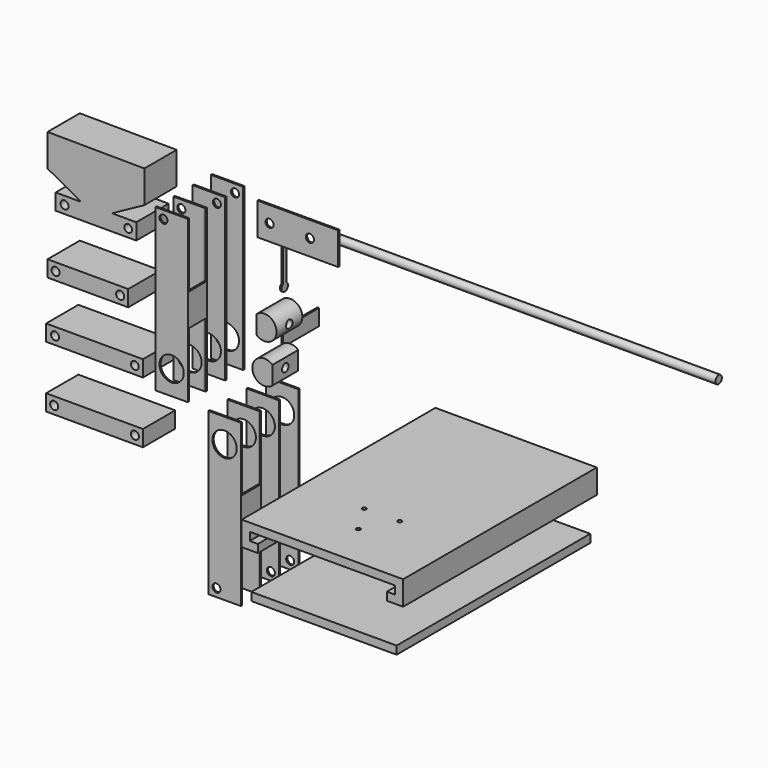
from build123d import *

# Parameters (mm, degrees)
F1_DEPTH  = 100
F2_R      = 7.5
F2_R_2    = 2.5
F3_DEPTH  = 15.001
F4_W      = 13
F4_H      = 40
F5_DEPTH  = 20.1627097718
F6_DEPTH  = 100
F7_R      = 7.5
F7_R_2    = 2.5
F8_DEPTH  = 16.001
F9_W      = 14
F9_H      = 40
F10_DEPTH = 20.1691592966
F11_W     = 50
F11_H     = 20
F11_R     = 2.5
F12_DEPTH = 1
F13_R     = 2.5
F13_R_2   = 7.5
F14_DEPTH = 45.1330833913
F15_R     = 7.5
F15_R_2   = 2.5
F16_DEPTH = 46.1330833913
F17_W     = 14
F17_H     = 40
F18_DEPTH = 53.5847666336
F19_W     = 13
F19_H     = 40
F20_DEPTH = 25
F22_DEPTH = 20
F23_R     = 2.5
F24_DEPTH = 250
F25_W     = 50
F25_H     = 10
F25_R     = 2.5
F26_DEPTH = 25
F25_R_2   = 2.4144593705
F25_W_2   = 60
F27_DEPTH = 25
F28_R     = 2.5
F29_DEPTH = 136.2251037518
F30_R     = 2.5
F31_DEPTH = 214.5146418358
F33_DEPTH = 1
F34_W     = 1
F34_H     = 10
F35_DEPTH = 25
F37_DEPTH = 150
F38_R     = 1.25
F39_DEPTH = 94.0357944536


# Not quite as in the source:
# - a feature names something its author has since deleted; it is built from what else it names


with BuildPart() as f1:
    # F0 (on Top) → F1 (new body)
    with BuildSketch(Plane.XY):
        Polygon((0, 14), (0, 15), (-20, 15), (-20, 0), (0, 0), (0, 1), (-19, 1), (-19, 14), align=None)
    extrude(amount=F1_DEPTH)

    # F2 (on face) → F3 (cut, through all)
    with BuildSketch(Plane.XZ):
        with Locations((-10, 15)):
            Circle(F2_R)
        with Locations((-5, 95)):
            Circle(F2_R_2)
    extrude(amount=-F3_DEPTH, mode=Mode.SUBTRACT)

    # F4 (on face) → F5 (cut, through all)
    with BuildSketch(Plane(origin=(-20, 0, 0), x_dir=(0, -1, 0), z_dir=(-1, 0, 0))):
        with Locations((-7.5, 20)):
            Rectangle(F4_W, F4_H)
        with Locations((-7.5, 80)):
            Rectangle(F4_W, F4_H)
    extrude(amount=-F5_DEPTH, mode=Mode.SUBTRACT)


with BuildPart() as f1b:
    # F0 (on Top) → F1, piece 2 (new body)
    with BuildSketch(Plane.XY):
        Polygon((0.051417134, -13.985459061), (-19.9480422158, -14.1325159114), (-19.9406893732, -15.1324888789), (-0.941202991, -14.992784871), (-0.8456160382, -27.9924334484), (-19.837749578, -28.1320833905), (-19.837749578, -29.1321104238), (0.1617097718, -28.9850535734), align=None)
    extrude(amount=F1_DEPTH)

    # F13 (on face) → F14 (cut, through all)
    with BuildSketch(Plane(origin=(0.2131255159, -28.9846755113, 0), x_dir=(0.9999729675, 0.0073528425, 0), z_dir=(0.0073528425, -0.9999729675, 0))):
        with Locations((-15.051417134, 95)):
            Circle(F13_R)
        with Locations((-10.051417134, 15)):
            Circle(F13_R_2)
    extrude(amount=-F14_DEPTH, mode=Mode.SUBTRACT)

    # F19 (on face) → F20 (cut)
    with BuildSketch(Plane(origin=(-0.0514157441, -0.0003780621, 0), x_dir=(-0.0073528425, 0.9999729675, 0), z_dir=(0.9999729675, 0.0073528425, 0))):
        with Locations((-21.485459061, 20)):
            Rectangle(F19_W, F19_H)
        with Locations((-21.485459061, 80)):
            Rectangle(F19_W, F19_H)
    extrude(amount=-F20_DEPTH, mode=Mode.SUBTRACT)


with BuildPart() as f6:
    # F0 (on Top) → F6 (new body)
    with BuildSketch(Plane.XY):
        Polygon((33.4159745649, 0), (33.4159745649, 1), (14.4159745649, 1), (14.4159745649, 15), (33.4159745649, 15), (33.4159745649, 16), (13.4159745649, 16), (13.4159745649, 0), align=None)
    extrude(amount=-F6_DEPTH)

    # F7 (on face) → F8 (cut, through all)
    with BuildSketch(Plane.XZ):
        with Locations((23.4159745649, -15)):
            Circle(F7_R)
        with Locations((28.4159745649, -95)):
            Circle(F7_R_2)
    extrude(amount=-F8_DEPTH, mode=Mode.SUBTRACT)

    # F9 (on face) → F10 (cut, through all)
    with BuildSketch(Plane(origin=(13.4159745649, 0, 0), x_dir=(0, -1, 0), z_dir=(-1, 0, 0))):
        with Locations((-8, -20)):
            Rectangle(F9_W, F9_H)
        with Locations((-8, -80)):
            Rectangle(F9_W, F9_H)
    extrude(amount=-F10_DEPTH, mode=Mode.SUBTRACT)


with BuildPart() as f6b:
    # F0 (on Top) → F6, piece 2 (new body)
    with BuildSketch(Plane.XY):
        Polygon((33.4664883811, -13.7397566624), (13.4670290313, -13.8868135128), (13.4743818739, -14.8867864803), (32.4738682561, -14.7470824724), (32.5768080514, -28.7467040172), (13.5846745117, -28.8863539594), (13.5846745117, -29.8863809926), (33.5841338614, -29.7393241422), align=None)
    extrude(amount=-F6_DEPTH)

    # F15 (on face) → F16 (cut, through all)
    with BuildSketch(Plane(origin=(0.2204783584, -29.9846484788, 0), x_dir=(0.9999729675, 0.0073528425, 0), z_dir=(0.0073528425, -0.9999729675, 0))):
        with Locations((23.3645574309, -15)):
            Circle(F15_R)
        with Locations((18.3645574309, -95)):
            Circle(F15_R_2)
    extrude(amount=-F16_DEPTH, mode=Mode.SUBTRACT)

    # F17 (on face) → F18 (cut, through all)
    with BuildSketch(Plane(origin=(33.3636555031, 0.2453243365, 0), x_dir=(-0.0073528425, 0.9999729675, 0), z_dir=(0.9999729675, 0.0073528425, 0))):
        with Locations((-21.985459061, -20)):
            Rectangle(F17_W, F17_H)
        with Locations((-21.985459061, -80)):
            Rectangle(F17_W, F17_H)
    extrude(amount=-F18_DEPTH, mode=Mode.SUBTRACT)


with BuildPart() as f12:
    # F11 (on Front) → F12 (new body)
    with BuildSketch(Plane.XZ):
        with Locations((45.8931141218, 95.3558683395)):
            Rectangle(F11_W, F11_H)
        with Locations((28.3931141218, 95.3558683395)):
            Circle(F11_R, mode=Mode.SUBTRACT)
        with Locations((53.3931141218, 95.3558683395)):
            Circle(F11_R, mode=Mode.SUBTRACT)
    extrude(amount=F12_DEPTH)


with BuildPart() as f22:
    # F21 (on Front) → F22 (new body)
    with BuildSketch(Plane.XZ):
        with BuildLine():
            Line((35.4863581642, 55.8813297105), (35.4863581642, 44.6073331245))
            ThreePointArc((35.4863581642, 44.6073331245), (47.9335038306, 50.2443314175), (35.4863581642, 55.8813297105))
        make_face()
    extrude(amount=F22_DEPTH)

    # F30 (on face) → F31 (cut, through all)
    with BuildSketch(Plane(origin=(35.4863581642, 0, 0), x_dir=(0, -1, 0), z_dir=(-1, 0, 0))):
        with Locations((10, 50.2443314175)):
            Circle(F30_R)
    extrude(amount=-F31_DEPTH, mode=Mode.SUBTRACT)


with BuildPart() as f22b:
    # F21 (on Front) → F22, piece 2 (new body)
    with BuildSketch(Plane.XZ):
        with BuildLine():
            Line((45.380649497, 20.1312099156), (45.380649497, 31.4052065016))
            ThreePointArc((45.380649497, 31.4052065016), (32.9335038306, 25.7682082086), (45.380649497, 20.1312099156))
        make_face()
    extrude(amount=F22_DEPTH)

    # F28 (on face) → F29 (cut, through all)
    with BuildSketch(Plane.YZ.offset(45.380649497)):
        with Locations((-10, 25.7682082086)):
            Circle(F28_R)
    extrude(amount=-F29_DEPTH, mode=Mode.SUBTRACT)


with BuildPart() as f24:
    # F23 (on Right) → F24 (new body)
    with BuildSketch(Plane.YZ):
        with Locations((69.883659482, 53.4276850522)):
            Circle(F23_R)
    extrude(amount=F24_DEPTH)


with BuildPart() as f26:
    # F25 (on Front) → F26 (new body)
    with BuildSketch(Plane.XZ):
        with Locations((-64.9493469292, 42.0624911785)):
            Rectangle(F25_W, F25_H)
        with Locations((-84.9493469292, 42.0624911785)):
            Circle(F25_R, mode=Mode.SUBTRACT)
        with Locations((-44.9493469292, 42.0624911785)):
            Circle(F25_R, mode=Mode.SUBTRACT)
    extrude(amount=F26_DEPTH)


with BuildPart() as f26b:
    # F25 (on Front) → F26, piece 2 (new body)
    with BuildSketch(Plane.XZ):
        Polygon((-84.9493469292, 85.124527216), (-84.9493469292, 75.124527216), (-34.9493469292, 75.124527216), (-34.9493469292, 85.124527216), (-49.9493469292, 85.124527216), (-29.9493469292, 96.0841532387), (-29.9493469292, 116.0841532387), (-89.9493469292, 116.5234603324), (-89.9493469292, 96.5234603324), (-69.9493469292, 85.5638343096), (-69.9493469292, 85.124527216), align=None)
        with Locations((-79.3778774142, 80.124527216)):
            Circle(F25_R, mode=Mode.SUBTRACT)
        with Locations((-39.9493469292, 80.124527216)):
            Circle(F25_R_2, mode=Mode.SUBTRACT)
    extrude(amount=F26_DEPTH)


with BuildPart() as f27:
    # F25 (on Front) → F27 (new body)
    with BuildSketch(Plane.XZ):
        with Locations((-60.8434542548, -31.3186603598)):
            Rectangle(F25_W_2, F25_H)
        with Locations((-85.8434542548, -31.3186603598)):
            Circle(F25_R, mode=Mode.SUBTRACT)
        with Locations((-35.8434542548, -31.3186603598)):
            Circle(F25_R, mode=Mode.SUBTRACT)
    extrude(amount=F27_DEPTH)


with BuildPart() as f27b:
    # F25 (on Front) → F27, piece 2 (new body)
    with BuildSketch(Plane.XZ):
        with Locations((-60.8434542548, 6.7433756776)):
            Rectangle(F25_W_2, F25_H)
        with Locations((-85.2719847398, 6.7433756776)):
            Circle(F25_R, mode=Mode.SUBTRACT)
        with Locations((-35.8434542548, 6.7433756776)):
            Circle(F25_R_2, mode=Mode.SUBTRACT)
    extrude(amount=F27_DEPTH)


with BuildPart() as f33:
    # F32 (on Right) → F33 (new body)
    with BuildSketch(Plane.YZ):
        with BuildLine():
            Line((47.762863338, 8.6800148711), (47.762863338, 20.4667558931))
            ThreePointArc((47.762863338, 20.4667558931), (46.3052242994, 24.9978365004), (44.8475852609, 20.4667558931))
            Line((44.8475852609, 20.4667558931), (44.8475852609, 8.6800148711))
            Line((44.8475852609, 8.6800148711), (44.8475852609, 0))
            Line((44.8475852609, 0), (47.762863338, 0))
            Line((47.762863338, 0), (47.762863338, 8.6800148711))
        make_face()
    extrude(amount=-F33_DEPTH)

    # F34 (on face) → F35 (join)
    with BuildSketch(Plane(origin=(0, 47.762863338, 0), x_dir=(-1, 0, 0), z_dir=(0, 1, 0))):
        with Locations((0.5, 5)):
            Rectangle(F34_W, F34_H)
    extrude(amount=F35_DEPTH)


with BuildPart() as f33b:
    # F32 (on Right) → F33, piece 2 (new body)
    with BuildSketch(Plane.YZ):
        with BuildLine():
            ThreePointArc((44.8475852609, 34.1576339639), (46.3052242994, 29.6265533566), (47.762863338, 34.1576339639))
            Line((47.762863338, 34.1576339639), (47.762863338, 45.944374986))
            Line((47.762863338, 45.944374986), (47.762863338, 54.6243898571))
            Line((47.762863338, 54.6243898571), (44.8475852609, 54.6243898571))
            Line((44.8475852609, 54.6243898571), (44.8475852609, 45.944374986))
            Line((44.8475852609, 45.944374986), (44.8475852609, 34.1576339639))
        make_face()
    extrude(amount=-F33_DEPTH)


with BuildPart() as f37:
    # F36 (on Front) → F37 (new body)
    with BuildSketch(Plane.XZ):
        Polygon((220.3795283456, 17.4886658788), (220.3795283456, 12.4886658788), (230.3795283456, 12.4886658788), (230.3795283456, 27.4886658788), (180.3795283456, 27.4886658788), (130.3795283456, 27.4886658788), (130.3795283456, 12.4886658788), (140.3795283456, 12.4886658788), (140.3795283456, 17.4886658788), (135.3795283456, 17.4886658788), (135.3795283456, 22.4886658788), (180.3795283456, 22.4886658788), (225.3795283456, 22.4886658788), (225.3795283456, 17.4886658788), align=None)
    extrude(amount=F37_DEPTH)

    # F38 (on face) → F39 (cut, through all)
    with BuildSketch(Plane(origin=(0, 0, 22.4886658788), x_dir=(1, 0, 0), z_dir=(0, 0, -1))):
        with Locations((180.5873862401, 122.4982716843)):
            Circle(F38_R)
        with Locations((169.4517786162, 103.9308743749)):
            Circle(F38_R)
        with Locations((191.0994201803, 103.5708539408)):
            Circle(F38_R)
    extrude(amount=-F39_DEPTH, mode=Mode.SUBTRACT)


with BuildPart() as f37b:
    # F36 (on Front) → F37, piece 2 (new body)
    with BuildSketch(Plane.XZ):
        Polygon((136.3347970862, -15.0014664978), (181.3347970862, -15.0014664978), (226.3347970862, -15.0014664978), (226.3347970862, -10.0014664978), (181.3347970862, -10.0014664978), (136.3347970862, -10.0014664978), align=None)
    extrude(amount=F37_DEPTH)


solid = Compound([f1.part, f1b.part, f6.part, f6b.part, f12.part, f22.part, f22b.part, f24.part, f26.part, f26b.part, f27.part, f27b.part, f33.part, f33b.part, f37.part, f37b.part])
